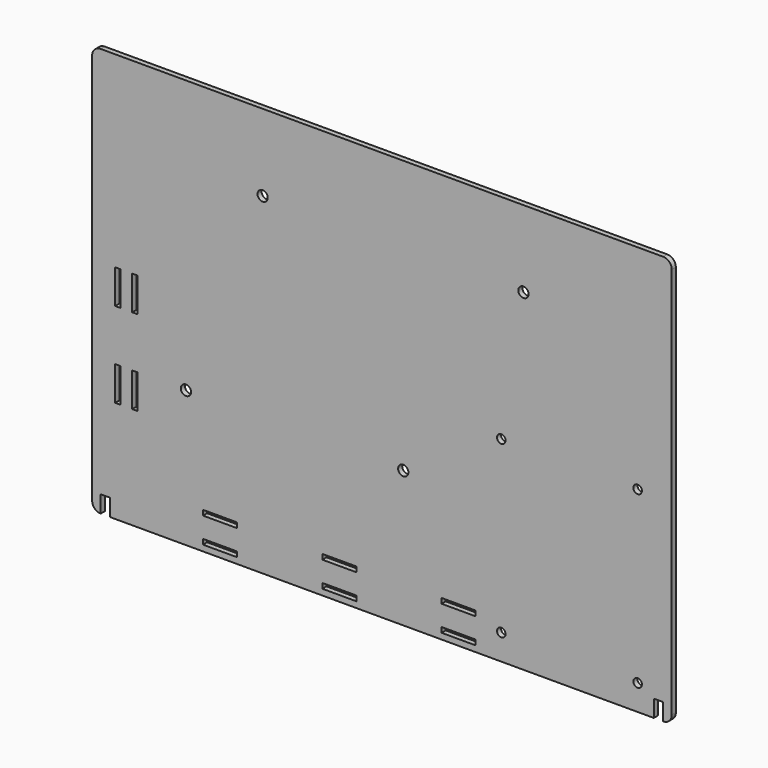
from build123d import *

# Parameters (mm, degrees)
F1_DEPTH = 3
F2_R     = 3
F3_DEPTH = 3
F4_R     = 2.5
F5_DEPTH = 3
F6_W     = 20
F6_H     = 3
F6_W_2   = 3
F6_H_2   = 20
F7_DEPTH = 3
F8_R     = 4.99999


# Not quite as in the source:
# - a fillet or chamfer is up to 0.001 mm smaller than in the source, because OpenCascade refuses the exact size


with BuildPart() as f1:
    # F0 (on Front) → F1 (new body)
    with BuildSketch(Plane.XZ):
        Polygon((165, -120), (170, -120), (170, 120), (-170, 120), (-170, -120), (-165, -120), (-165, -110), (-159.5, -110), (-159.5, -120), (159.5, -120), (159.5, -110), (165, -110), align=None)
    extrude(amount=F1_DEPTH)

    # F2 (on face) → F3 (cut, through all)
    with BuildSketch(Plane.XZ.offset(3)):
        with Locations((-70, 75)):
            Circle(F2_R)
        with Locations((83, 75)):
            Circle(F2_R)
        with Locations((12.5, -40)):
            Circle(F2_R)
        with Locations((-115, -40)):
            Circle(F2_R)
    extrude(amount=-F3_DEPTH, mode=Mode.SUBTRACT)

    # F4 (on face) → F5 (cut, through all)
    with BuildSketch(Plane.XZ.offset(3)):
        with Locations((70, -5)):
            Circle(F4_R)
        with Locations((150, -5)):
            Circle(F4_R)
        with Locations((150, -105)):
            Circle(F4_R)
        with Locations((70, -105)):
            Circle(F4_R)
    extrude(amount=-F5_DEPTH, mode=Mode.SUBTRACT)

    # F6 (on face) → F7 (cut, through all)
    with BuildSketch(Plane.XZ.offset(3)):
        with Locations((-95, -100)):
            Rectangle(F6_W, F6_H)
        with Locations((-25, -100)):
            Rectangle(F6_W, F6_H)
        with Locations((45, -100)):
            Rectangle(F6_W, F6_H)
        with Locations((-95, -115)):
            Rectangle(F6_W, F6_H)
        with Locations((-25, -115)):
            Rectangle(F6_W, F6_H)
        with Locations((45, -115)):
            Rectangle(F6_W, F6_H)
        with Locations((-155, 0)):
            Rectangle(F6_W_2, F6_H_2)
        with Locations((-145, 0)):
            Rectangle(F6_W_2, F6_H_2)
        with Locations((-155, -50)):
            Rectangle(F6_W_2, F6_H_2)
        with Locations((-145, -50)):
            Rectangle(F6_W_2, F6_H_2)
    extrude(amount=-F7_DEPTH, mode=Mode.SUBTRACT)

    # F8 (radius 5 in the source; OpenCascade refuses exactly that, so slightly less here)
    f8_edges = [f1.edges().sort_by_distance(p)[0] for p in [
        (-170, -1.5, 120),
        (170, -1.5, 120),
        (170, -1.5, -120),
        (-170, -1.5, -120),
    ]]
    fillet(f8_edges, radius=F8_R)


solid = f1.part
